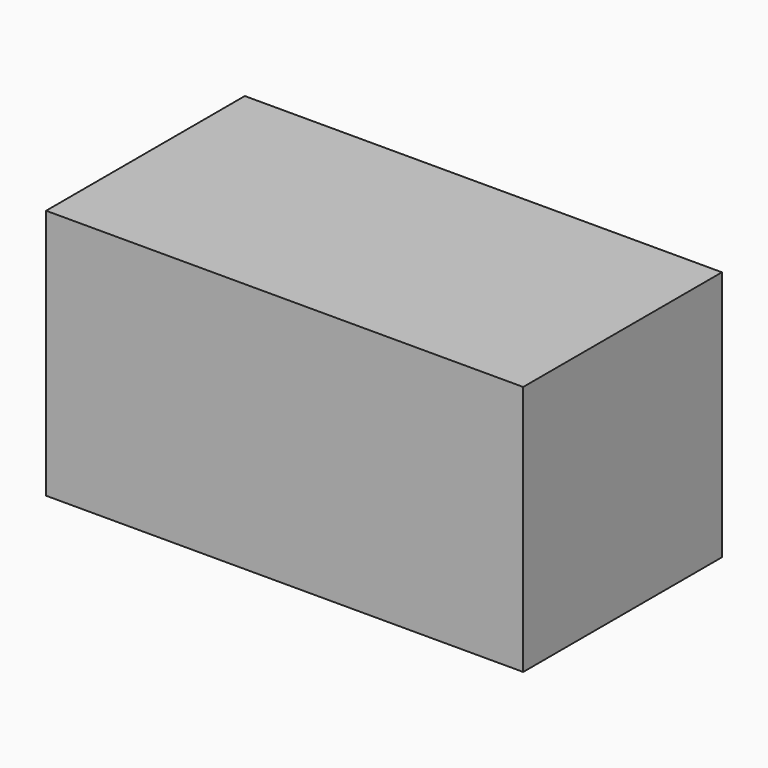
from build123d import *

# Parameters (mm, degrees)
F0_W     = 95.0807929039
F0_H     = 49.5008267462
F1_DEPTH = 50


# Not quite as in the source:
# - the program builds the solid bodies; features that only make, move or delete a surface that nothing else refers to are left out


with BuildPart() as f1:
    # F0 (on Top) → F1 (new body)
    with BuildSketch(Plane.XY):
        with Locations((0.4901066422, -2.0829550922)):
            Rectangle(F0_W, F0_H)
    extrude(amount=F1_DEPTH)


solid = f1.part
